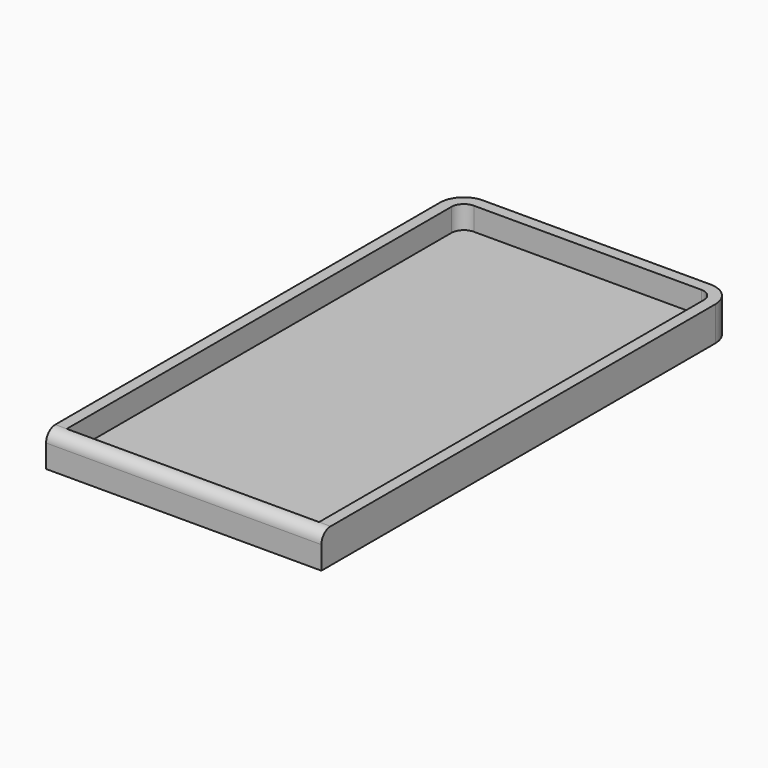
from build123d import *

# Parameters (mm, degrees)
F1_DEPTH = 9
F2_T     = -3
F3_R     = 2.99999


# Not quite as in the source:
# - a fillet or chamfer is up to 0.001 mm smaller than in the source, because OpenCascade refuses the exact size


with BuildPart() as f1:
    # F0 (on Top) → F1 (new body)
    with BuildSketch(Plane.XY):
        with BuildLine():
            Line((-74.3585927405, 75.2026882768), (-74.3585927405, -53.5473117232))
            Line((-74.3585927405, -53.5473117232), (-2.3585927405, -53.5473117232))
            Line((-2.3585927405, -53.5473117232), (-2.3585927405, 75.2026882768))
            ThreePointArc((-2.3585927405, 75.2026882768), (-4.189175358, 79.6221056592), (-8.6085927405, 81.4526882768))
            Line((-8.6085927405, 81.4526882768), (-68.1085927405, 81.4526882768))
            ThreePointArc((-68.1085927405, 81.4526882768), (-72.5280101229, 79.6221056592), (-74.3585927405, 75.2026882768))
        make_face()
    extrude(amount=F1_DEPTH)

    # F2
    f2_openings = [f1.faces().sort_by_distance(p)[0] for p in [
        (-38.358593, 13.83847, 9),
    ]]
    offset(amount=F2_T, openings=f2_openings)

    # F3 (radius 3 in the source; OpenCascade refuses exactly that, so slightly less here)
    f3_edges = [f1.edges().sort_by_distance(p)[0] for p in [
        (-38.358593, -53.547312, 9),
    ]]
    fillet(f3_edges, radius=F3_R)


solid = f1.part
